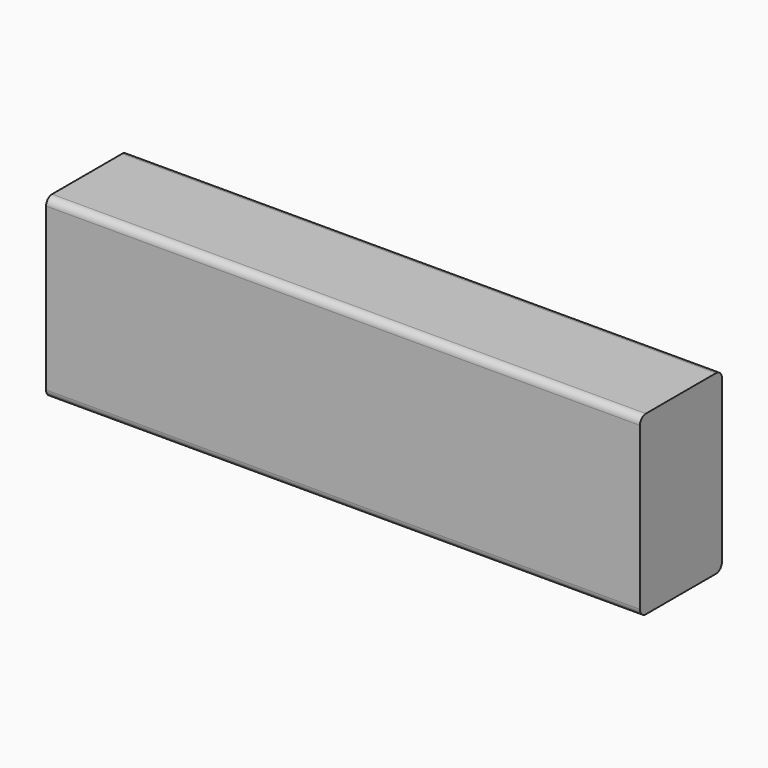
from build123d import *

# Parameters (mm, degrees)
F0_W     = 17.526
F0_H     = 30.226
F1_DEPTH = 101.6
F2_W     = 2.54
F2_H     = 30.226
F3_DEPTH = 0.127
F4_R     = 1.2699


# Not quite as in the source:
# - a fillet or chamfer is up to 0.001 mm smaller than in the source, because OpenCascade refuses the exact size


with BuildPart() as f1:
    # F0 (on Right) → F1 (new body)
    with BuildSketch(Plane.YZ):
        with Locations((-9.1045090495, 12.8600424648)):
            Rectangle(F0_W, F0_H)
    extrude(amount=F1_DEPTH)

    # F2 (on face) → F3 (cut)
    with BuildSketch(Plane(origin=(0, -0.3415090495, 0), x_dir=(-1, 0, 0), z_dir=(0, 1, 0))):
        with Locations((-52.07, 12.8600424648)):
            Rectangle(F2_W, F2_H)
    extrude(amount=-F3_DEPTH, mode=Mode.SUBTRACT)

    # F4 (radius 1.27 in the source; OpenCascade refuses exactly that, so slightly less here)
    f4_edges = [f1.edges().sort_by_distance(p)[0] for p in [
        (77.47, -0.341509, 27.973042),
        (50.8, -17.867509, 27.973042),
        (50.8, -17.867509, -2.252958),
        (25.4, -0.341509, -2.252958),
    ]]
    fillet(f4_edges, radius=F4_R)


solid = f1.part
